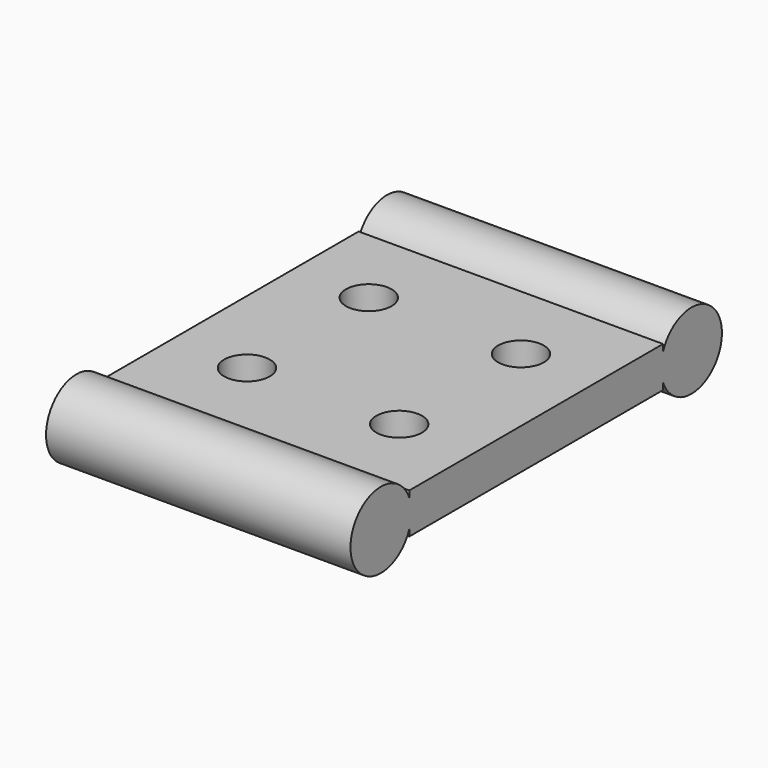
from build123d import *

# Parameters (mm, degrees)
F0_W     = 60
F0_H     = 62.5
F1_DEPTH = 8
F3_D     = 9
F3_DEPTH = 15
F3_TIP   = 2.7038727856
F5_DEPTH = 60


with BuildPart() as f1:
    # F0 (on Top) → F1 (new body)
    with BuildSketch(Plane.XY):
        with Locations((30, -31.25)):
            Rectangle(F0_W, F0_H)
    extrude(amount=F1_DEPTH)

    # F3
    with Locations(Plane.XY.offset(8)):
        with Locations((15, -16.25), (45, -16.25), (45, -46.25), (15, -46.25)):
            Hole(F3_D / 2, depth=F3_DEPTH)
            with Locations((0, 0, -(F3_DEPTH + F3_TIP / 2))):  # 118° drill point
                Cone(0, F3_D / 2, F3_TIP, mode=Mode.SUBTRACT)

    # F4 (on face) → F5 (join)
    with BuildSketch(Plane.YZ.offset(60)):
        with BuildLine():
            ThreePointArc((-62.5, 1.3074175964), (-62.1260593981, 2.6306936062), (-62, 4))
            ThreePointArc((-62, 4), (-62.1260593981, 5.3693063938), (-62.5, 6.6925824036))
            Line((-62.5, 6.6925824036), (-62.5, 1.3074175964))
        make_face()
        with BuildLine():
            Line((-62.5, 1.3074175964), (-62.5, 6.6925824036))
            ThreePointArc((-62.5, 6.6925824036), (-77, 4), (-62.5, 1.3074175964))
        make_face()
        with BuildLine():
            ThreePointArc((14.5, 4), (8.3693063938, 11.3739406019), (0, 6.6925824036))
            Line((0, 6.6925824036), (0, 1.3074175964))
            ThreePointArc((0, 1.3074175964), (8.3693063938, -3.3739406019), (14.5, 4))
        make_face()
    extrude(amount=-F5_DEPTH)


solid = f1.part
